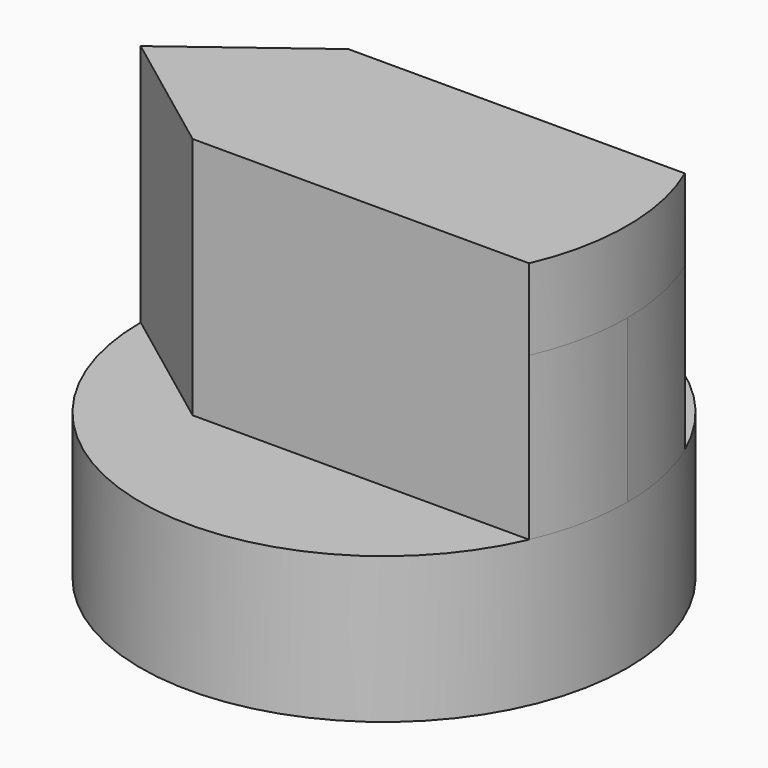
from build123d import *

# Parameters (mm, degrees)
F0_R     = 15
F1_DEPTH = 9
F2_R     = 0.5
F3_DEPTH = 10
F6_DEPTH = 5


# Not quite as in the source:
# - a fillet or chamfer that OpenCascade refuses, or shapes differently, is made with other operations: its cross-section is extruded or revolved along the edge and cut away or added


with BuildPart() as f1:
    # F0 (on Top) → F1 (new body)
    with BuildSketch(Plane.XY):
        Circle(F0_R)
        with BuildLine():
            Line((-2.2, -2.3237900077), (-2.2, 2.3237900077))
            ThreePointArc((-2.2, 2.3237900077), (3.2, 0), (-2.2, -2.3237900077))
        make_face(mode=Mode.SUBTRACT)
    extrude(amount=F1_DEPTH)

    # F2 (on face) → F3 (join)
    with BuildSketch(Plane.XY.offset(9)):
        with BuildLine():
            Line((-7, 6), (-15, 0))
            Line((-15, 0), (-7, -6))
            Line((-7, -6), (13.7477270849, -6))
            ThreePointArc((13.7477270849, -6), (14.683594694, -3.0646446553), (15, 0))
            ThreePointArc((15, 0), (14.683594694, 3.0646446553), (13.7477270849, 6))
            Line((13.7477270849, 6), (-7, 6))
        make_face()
        Circle(F2_R, mode=Mode.SUBTRACT)
    extrude(amount=F3_DEPTH)

    # F4: chamfer of 10 x 2.6794919243 on 1 edges, made by hand


with BuildPart() as f4_tool2:
    # F4_s3 → F4_t4 (revolve)
    with BuildSketch(Plane.XZ):
        Polygon((3.1794919243, 9), (0.5, 19), (0.5, 9), align=None)
    revolve(axis=Axis((0, 0, 9), (0, 0, 1)))

    split(bisect_by=Plane.YZ.offset(-2.2), keep=Keep.TOP)


with BuildPart() as f1_1:
    add(f1.part)

    # F4_t1: cut F4_tool2
    add(f4_tool2.part, mode=Mode.SUBTRACT)

    # F5 (on face) → F6 (join)
    with BuildSketch(Plane.XY.offset(19)):
        with BuildLine():
            Line((-7, 6), (-15, 0))
            Line((-15, 0), (-7, -6))
            Line((-7, -6), (13.7477270849, -6))
            ThreePointArc((13.7477270849, -6), (15, 0), (13.7477270849, 6))
            Line((13.7477270849, 6), (-7, 6))
        make_face()
    extrude(amount=F6_DEPTH)


solid = f1_1.part
